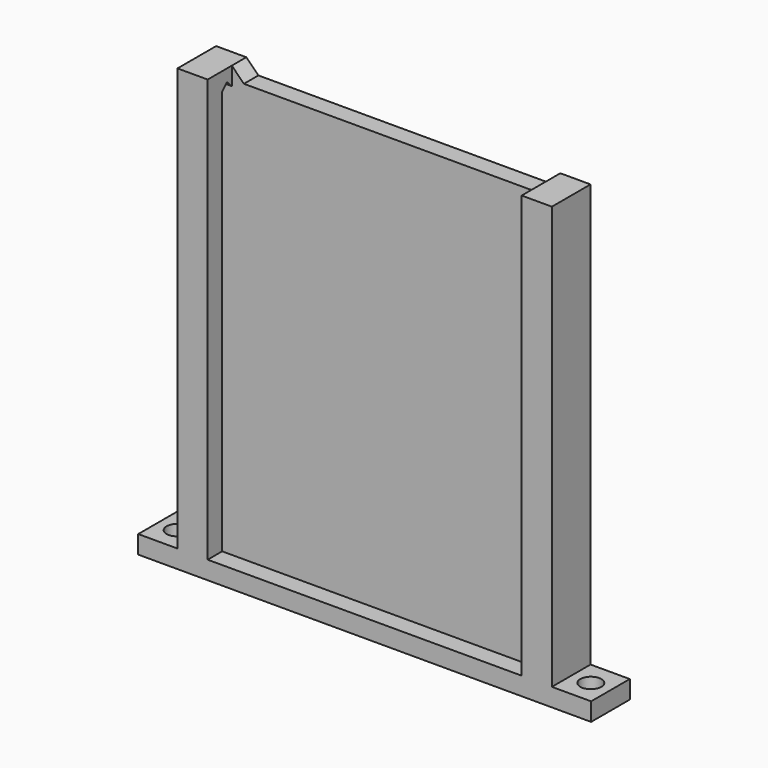
from build123d import *

# Parameters (mm, degrees)
F0_W     = 75
F0_H     = 8
F0_R     = 1.75
F0_W_2   = 56
F0_H_2   = 2
F1_DEPTH = 3
F3_DEPTH = 68
F4_W     = 5
F4_H     = 8
F5_DEPTH = 2
F6_SIZE  = 1.99999
F7_SIZE  = 0.99999
F8_SIZE  = 0.5


# Not quite as in the source:
# - a fillet or chamfer is up to 0.001 mm smaller than in the source, because OpenCascade refuses the exact size


with BuildPart() as f1:
    # F0 (on Top) → F1 (new body)
    with BuildSketch(Plane.XY):
        Rectangle(F0_W, F0_H)
        with Locations((-34.25, 0)):
            Circle(F0_R, mode=Mode.SUBTRACT)
        Rectangle(F0_W_2, F0_H_2, mode=Mode.SUBTRACT)
        with Locations((34.25, 0)):
            Circle(F0_R, mode=Mode.SUBTRACT)
    extrude(amount=F1_DEPTH)

    # F2 (on face) → F3 (join)
    with BuildSketch(Plane.XY.offset(3)):
        Polygon((-31, 4), (-31, -4), (-26, -4), (-26, -1), (-28, -1), (-28, 1), (28, 1), (28, -1), (26, -1), (26, -4), (31, -4), (31, 4), align=None)
    extrude(amount=F3_DEPTH)

    # F4 (on face) → F5 (join)
    with BuildSketch(Plane.XY.offset(71)):
        with Locations((-28.5, 0)):
            Rectangle(F4_W, F4_H)
        with Locations((28.5, 0)):
            Rectangle(F4_W, F4_H)
    extrude(amount=F5_DEPTH)

    # F6 (size 2 in the source; OpenCascade refuses exactly that, so slightly less here)
    f6_edges = [f1.edges().sort_by_distance(p)[0] for p in [
        (-26, 2.5, 71),
        (26, 2.5, 71),
    ]]
    chamfer(f6_edges, length=F6_SIZE)

    # F7 (size 1 in the source; OpenCascade refuses exactly that, so slightly less here)
    f7_edges = [f1.edges().sort_by_distance(p)[0] for p in [
        (-27, 1, 71),
        (27, 1, 71),
        (27, -1, 71),
        (-27, -1, 71),
    ]]
    chamfer(f7_edges, length=F7_SIZE)

    # F8
    f8_edges = [f1.edges().sort_by_distance(p)[0] for p in [
        (0, -1, 0),
        (0, 1, 0),
        (-28, 0, 0),
        (28, 0, 0),
    ]]
    chamfer(f8_edges, length=F8_SIZE)


solid = f1.part
